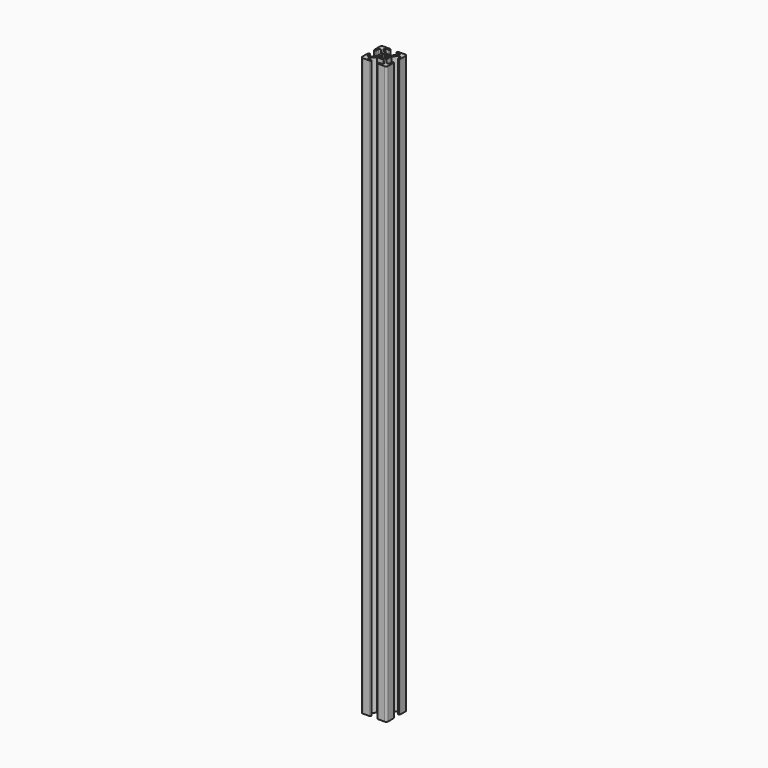
from build123d import *

# Parameters (mm, degrees)
F1_DEPTH = 11430


# Not quite as in the source:
# - ends of sketch curves that miss each other by under 0.0002 mm in the source are joined


with BuildPart() as f1:
    # F0 (on Top) → F1 (new body)
    with BuildSketch(Plane.XY):
        with BuildLine():
            Line((228.8032, 66.802), (241.0968, 66.802))
            ThreePointArc((241.0968, 66.802), (250.220740219, 70.581259781), (254, 79.7052))
            Line((254, 79.7052), (254, 215.9))
            ThreePointArc((254, 215.9), (242.8407683632, 242.8407683632), (215.9, 254))
            Line((215.9, 254), (79.7052, 254))
            ThreePointArc((79.7052, 254), (70.581259781, 250.220740219), (66.802, 241.0968))
            Line((66.802, 241.0968), (66.802, 228.8032))
            ThreePointArc((66.802, 228.8032), (70.581259781, 219.679259781), (79.7052, 215.9))
            Line((79.7052, 215.9), (139.3698, 215.9))
            ThreePointArc((139.3698, 215.9), (148.493740219, 212.120740219), (152.273, 202.9968))
            Line((152.273, 202.9968), (152.273, 184.5584574))
            ThreePointArc((152.273, 184.5584574), (151.2907989473, 179.6206082388), (148.493727519, 175.434504481))
            Line((148.493727519, 175.434504481), (69.675502, 96.616266))
            ThreePointArc((69.675502, 96.616266), (65.4893917612, 93.8192010527), (60.5515426, 92.837))
            Line((60.5515426, 92.837), (-60.5515426, 92.837))
            ThreePointArc((-60.5515426, 92.837), (-65.4893917612, 93.8192010527), (-69.675495519, 96.616272481))
            Line((-69.675495519, 96.616272481), (-148.493734, 175.434498))
            ThreePointArc((-148.493734, 175.434498), (-151.2907989473, 179.6206082388), (-152.273, 184.5584574))
            Line((-152.273, 184.5584574), (-152.273, 202.9968))
            ThreePointArc((-152.273, 202.9968), (-148.493740219, 212.120740219), (-139.3698, 215.9))
            Line((-139.3698, 215.9), (-79.7052, 215.9))
            ThreePointArc((-79.7052, 215.9), (-70.581259781, 219.679259781), (-66.802, 228.8032))
            Line((-66.802, 228.8032), (-66.802, 241.0968))
            ThreePointArc((-66.802, 241.0968), (-70.581259781, 250.220740219), (-79.7052, 254))
            Line((-79.7052, 254), (-215.9, 254))
            ThreePointArc((-215.9, 254), (-242.8407683632, 242.8407683632), (-254, 215.9))
            Line((-254, 215.9), (-254, 79.7052))
            ThreePointArc((-254, 79.7052), (-250.220740219, 70.581259781), (-241.0968, 66.802))
            Line((-241.0968, 66.802), (-228.8032, 66.802))
            ThreePointArc((-228.8032, 66.802), (-219.679259781, 70.581259781), (-215.9, 79.7052))
            Line((-215.9, 79.7052), (-215.9, 139.3698))
            ThreePointArc((-215.9, 139.3698), (-212.120740219, 148.493740219), (-202.9968, 152.273))
            Line((-202.9968, 152.273), (-184.5584574, 152.273))
            ThreePointArc((-184.5584574, 152.273), (-179.6206082388, 151.2907989473), (-175.434504481, 148.493727519))
            Line((-175.434504481, 148.493727519), (-96.616266, 69.675502))
            ThreePointArc((-96.616266, 69.675502), (-93.8192010527, 65.4893917612), (-92.837, 60.5515426))
            Line((-92.837, 60.5515426), (-92.837, -60.5515426))
            ThreePointArc((-92.837, -60.5515426), (-93.8192010527, -65.4893917612), (-96.616272481, -69.675495519))
            Line((-96.616272481, -69.675495519), (-175.434498, -148.493734))
            ThreePointArc((-175.434498, -148.493734), (-179.6206082388, -151.2907989473), (-184.5584574, -152.273))
            Line((-184.5584574, -152.273), (-202.9968, -152.273))
            ThreePointArc((-202.9968, -152.273), (-212.120740219, -148.493740219), (-215.9, -139.3698))
            Line((-215.9, -139.3698), (-215.9, -79.7052))
            ThreePointArc((-215.9, -79.7052), (-219.679259781, -70.581259781), (-228.8032, -66.802))
            Line((-228.8032, -66.802), (-241.0968, -66.802))
            ThreePointArc((-241.0968, -66.802), (-250.220740219, -70.581259781), (-254, -79.7052))
            Line((-254, -79.7052), (-254, -215.9))
            ThreePointArc((-254, -215.9), (-242.8407683632, -242.8407683632), (-215.9, -254))
            Line((-215.9, -254), (-79.7052, -254))
            ThreePointArc((-79.7052, -254), (-70.581259781, -250.220740219), (-66.802, -241.0968))
            Line((-66.802, -241.0968), (-66.802, -228.8032))
            ThreePointArc((-66.802, -228.8032), (-70.581259781, -219.679259781), (-79.7052, -215.9))
            Line((-79.7052, -215.9), (-139.3698, -215.9))
            ThreePointArc((-139.3698, -215.9), (-148.493740219, -212.120740219), (-152.273, -202.9968))
            Line((-152.273, -202.9968), (-152.273, -184.5584574))
            ThreePointArc((-152.273, -184.5584574), (-151.2907989473, -179.6206082388), (-148.493727519, -175.434504481))
            Line((-148.493727519, -175.434504481), (-69.675502, -96.616266))
            ThreePointArc((-69.675502, -96.616266), (-65.4893917612, -93.8192010527), (-60.5515426, -92.837))
            Line((-60.5515426, -92.837), (60.5515426, -92.837))
            ThreePointArc((60.5515426, -92.837), (65.4893917612, -93.8192010527), (69.675495519, -96.616272481))
            Line((69.675495519, -96.616272481), (148.493734, -175.434498))
            ThreePointArc((148.493734, -175.434498), (151.2907989473, -179.6206082388), (152.273, -184.5584574))
            Line((152.273, -184.5584574), (152.273, -202.9968))
            ThreePointArc((152.273, -202.9968), (148.493740219, -212.120740219), (139.3698, -215.9))
            Line((139.3698, -215.9), (79.7052, -215.9))
            ThreePointArc((79.7052, -215.9), (70.581259781, -219.679259781), (66.802, -228.8032))
            Line((66.802, -228.8032), (66.802, -241.0968))
            ThreePointArc((66.802, -241.0968), (70.581259781, -250.220740219), (79.7052, -254))
            Line((79.7052, -254), (215.9, -254))
            ThreePointArc((215.9, -254), (242.8407683632, -242.8407683632), (254, -215.9))
            Line((254, -215.9), (254, -79.7052))
            ThreePointArc((254, -79.7052), (250.220740219, -70.581259781), (241.0968, -66.802))
            Line((241.0968, -66.802), (228.8032, -66.802))
            ThreePointArc((228.8032, -66.802), (219.679259781, -70.581259781), (215.9, -79.7052))
            Line((215.9, -79.7052), (215.9, -139.3698))
            ThreePointArc((215.9, -139.3698), (212.120740219, -148.493740219), (202.9968, -152.273))
            Line((202.9968, -152.273), (184.5584574, -152.273))
            ThreePointArc((184.5584574, -152.273), (179.6206082388, -151.2907989473), (175.434504481, -148.493727519))
            Line((175.434504481, -148.493727519), (96.616266, -69.675502))
            ThreePointArc((96.616266, -69.675502), (93.8192010527, -65.4893917612), (92.837, -60.5515426))
            Line((92.837, -60.5515426), (92.837, 60.5515426))
            ThreePointArc((92.837, 60.5515426), (93.8192010527, 65.4893917612), (96.616272481, 69.675495519))
            Line((96.616272481, 69.675495519), (175.434498, 148.493734))
            ThreePointArc((175.434498, 148.493734), (179.6206082388, 151.2907989473), (184.5584574, 152.273))
            Line((184.5584574, 152.273), (202.9968, 152.273))
            ThreePointArc((202.9968, 152.273), (212.120740219, 148.493740219), (215.9, 139.3698))
            Line((215.9, 139.3698), (215.9, 79.7052))
            ThreePointArc((215.9, 79.7052), (219.679259781, 70.581259781), (228.8032, 66.802))
        make_face()
        with BuildLine():
            ThreePointArc((-20.4210161511, -49.152403514), (-34.4542925862, -63.6508288974), (-53.9724863346, -58.5344533346))
            Line((-53.9724863346, -58.5344533346), (-58.5344524, -53.9724854))
            ThreePointArc((-58.5344524, -53.9724854), (-63.6508288974, -34.4542925862), (-49.152403514, -20.4210161511))
            ThreePointArc((-49.152403514, -20.4210161511), (-53.2257, 0), (-49.1523903665, 20.421010302))
            ThreePointArc((-49.1523903665, 20.421010302), (-63.6508288974, 34.4542925862), (-58.5344533346, 53.9724863346))
            Line((-58.5344533346, 53.9724863346), (-53.9724854, 58.5344524))
            ThreePointArc((-53.9724854, 58.5344524), (-34.4542925862, 63.6508288974), (-20.4210161511, 49.152403514))
            ThreePointArc((-20.4210161511, 49.152403514), (0, 53.2257), (20.421010302, 49.1523903665))
            ThreePointArc((20.421010302, 49.1523903665), (34.4542925862, 63.6508288974), (53.9724863346, 58.5344533346))
            Line((53.9724863346, 58.5344533346), (58.5344524, 53.9724854))
            ThreePointArc((58.5344524, 53.9724854), (63.6508288974, 34.4542925862), (49.152403514, 20.4210161511))
            ThreePointArc((49.152403514, 20.4210161511), (53.2257, 0), (49.1523903665, -20.421010302))
            ThreePointArc((49.1523903665, -20.421010302), (63.6508288974, -34.4542925862), (58.5344533346, -53.9724863346))
            Line((58.5344533346, -53.9724863346), (53.9724854, -58.5344524))
            ThreePointArc((53.9724854, -58.5344524), (34.4542925862, -63.6508288974), (20.4210161511, -49.152403514))
            ThreePointArc((20.4210161511, -49.152403514), (0, -53.2257), (-20.4210161511, -49.152403514))
        make_face(mode=Mode.SUBTRACT)
    extrude(amount=F1_DEPTH)


solid = f1.part
